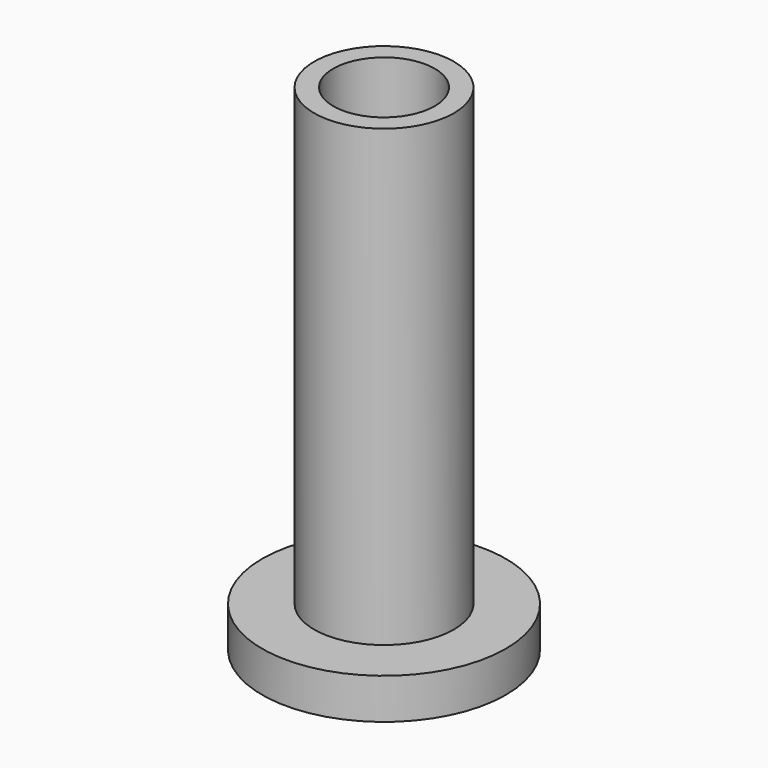
from build123d import *

# Parameters (mm, degrees)
F0_R     = 4.3688
F1_DEPTH = 28.4226
F0_R_2   = 7.62
F2_DEPTH = 2.54
F3_R     = 3.175
F4_DEPTH = 30.9636


# Not quite as in the source:
# - a feature names something its author has since deleted; it is built from what else it names


with BuildPart() as f1:
    # F0 (on Top) → F1 (new body)
    with BuildSketch(Plane.XY):
        Circle(F0_R)
    extrude(amount=F1_DEPTH)

    # F0 (on Top) → F2 (join)
    with BuildSketch(Plane.XY):
        Circle(F0_R_2)
        Circle(F0_R, mode=Mode.SUBTRACT)
        Circle(F0_R)
    extrude(amount=-F2_DEPTH)

    # F3 (on face) → F4 (cut, through all)
    with BuildSketch(Plane.XY.offset(28.4226)):
        Circle(F3_R)
    extrude(amount=-F4_DEPTH, mode=Mode.SUBTRACT)


solid = f1.part
